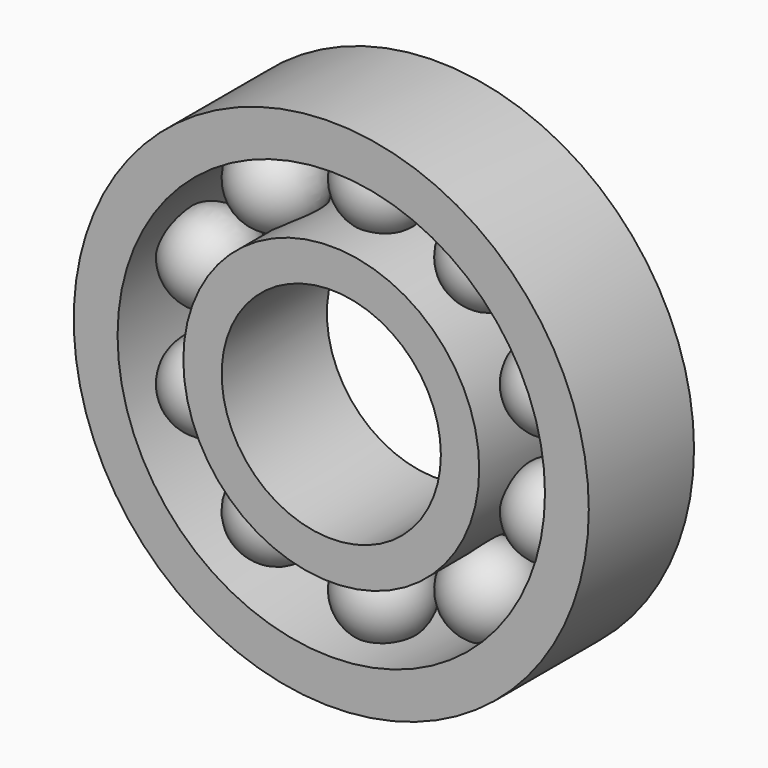
from build123d import *

# Parameters (mm, degrees)
F1_R     = 23.5
F1_R_2   = 19.5
F2_DEPTH = 12
F0_R     = 13.5
F0_R_2   = 10
F3_DEPTH = 12
F8_COUNT = 10


with BuildPart() as f2:
    # F1 (on Front) → F2 (new body)
    with BuildSketch(Plane.XZ):
        Circle(F1_R)
        Circle(F1_R_2, mode=Mode.SUBTRACT)
    extrude(amount=-F2_DEPTH)


with BuildPart() as f3:
    # F0 (on Front) → F3 (new body)
    with BuildSketch(Plane.XZ):
        Circle(F0_R)
        Circle(F0_R_2, mode=Mode.SUBTRACT)
    extrude(amount=-F3_DEPTH)


with BuildPart() as f6:
    # F5 (on offset) → F6 (revolve)
    with BuildSketch(Plane.XZ.offset(-6)):
        with BuildLine():
            Line((0, 20.5), (0, 12.5))
            ThreePointArc((0, 12.5), (4, 16.5), (0, 20.5))
        make_face()
    revolve(axis=Axis((0, 6, 16.5), (0, 0, 1)))


with BuildPart() as f8_1:
    # F8: instance of F6
    add(f6.part.rotate(Axis((0, -1.2231208384, 0), (0, 1, 0)), 1 * 360 / F8_COUNT))


with BuildPart() as f8_2:
    # F8: instance of F6
    add(f6.part.rotate(Axis((0, -1.2231208384, 0), (0, 1, 0)), 2 * 360 / F8_COUNT))


with BuildPart() as f8_3:
    # F8: instance of F6
    add(f6.part.rotate(Axis((0, -1.2231208384, 0), (0, 1, 0)), 3 * 360 / F8_COUNT))


with BuildPart() as f8_4:
    # F8: instance of F6
    add(f6.part.rotate(Axis((0, -1.2231208384, 0), (0, 1, 0)), 4 * 360 / F8_COUNT))


with BuildPart() as f8_5:
    # F8: instance of F6
    add(f6.part.rotate(Axis((0, -1.2231208384, 0), (0, 1, 0)), 5 * 360 / F8_COUNT))


with BuildPart() as f8_6:
    # F8: instance of F6
    add(f6.part.rotate(Axis((0, -1.2231208384, 0), (0, 1, 0)), 6 * 360 / F8_COUNT))


with BuildPart() as f8_7:
    # F8: instance of F6
    add(f6.part.rotate(Axis((0, -1.2231208384, 0), (0, 1, 0)), 7 * 360 / F8_COUNT))


with BuildPart() as f8_8:
    # F8: instance of F6
    add(f6.part.rotate(Axis((0, -1.2231208384, 0), (0, 1, 0)), 8 * 360 / F8_COUNT))


with BuildPart() as f8_9:
    # F8: instance of F6
    add(f6.part.rotate(Axis((0, -1.2231208384, 0), (0, 1, 0)), 9 * 360 / F8_COUNT))


solid = Compound([f2.part, f3.part, f6.part, f8_1.part, f8_2.part, f8_3.part, f8_4.part, f8_5.part, f8_6.part, f8_7.part, f8_8.part, f8_9.part])
